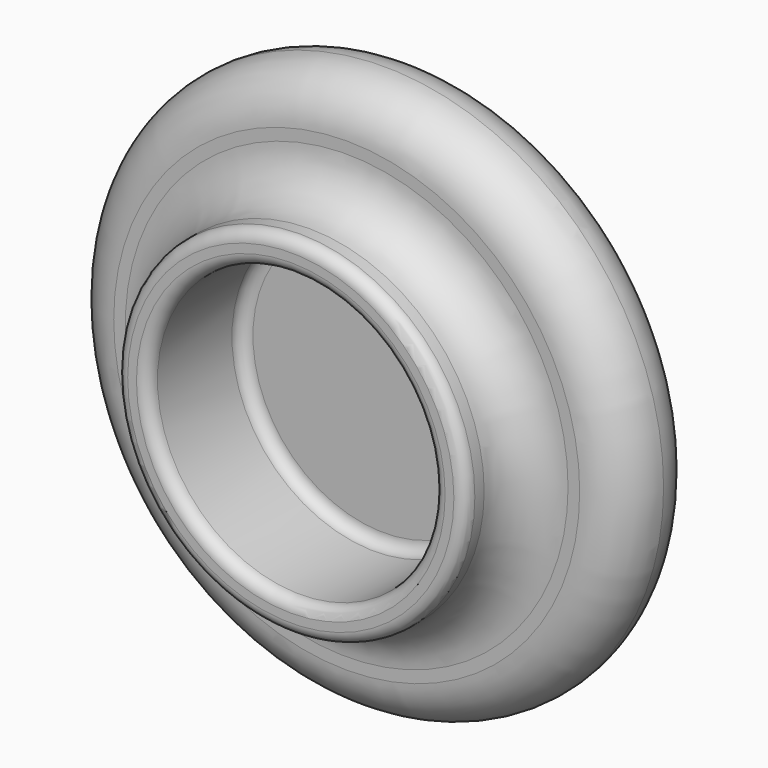
from build123d import *

# Parameters (mm, degrees)
F0_R     = 12
F0_R_2   = 7.5
F0_R_3   = 6.125
F1_DEPTH = 4
F2_DEPTH = 3
F3_DEPTH = 2
F4_R     = 1.99999
F5_R     = 0.5


# Not quite as in the source:
# - a fillet or chamfer is up to 0.001 mm smaller than in the source, because OpenCascade refuses the exact size


with BuildPart() as f1:
    # F0 (on Front) → F1 (new body)
    with BuildSketch(Plane.XZ):
        Circle(F0_R)
        Circle(F0_R_2, mode=Mode.SUBTRACT)
        Circle(F0_R_2)
        Circle(F0_R_3, mode=Mode.SUBTRACT)
        Circle(F0_R_3)
    extrude(amount=-F1_DEPTH)

    # F0 (on Front) → F2 (join)
    with BuildSketch(Plane.XZ):
        Circle(F0_R_2)
        Circle(F0_R_3, mode=Mode.SUBTRACT)
    extrude(amount=F2_DEPTH)

    # F0 (on Front) → F3 (cut)
    with BuildSketch(Plane.XZ):
        Circle(F0_R_3)
    extrude(amount=-F3_DEPTH, mode=Mode.SUBTRACT)

    # F4 (radius 2 in the source; OpenCascade refuses exactly that, so slightly less here)
    f4_edges = [f1.edges().sort_by_distance(p)[0] for p in [
        (-7.5, 0, 0),
        (-12, 0, 0),
        (-12, 4, 0),
    ]]
    fillet(f4_edges, radius=F4_R)

    # F5
    f5_edges = [f1.edges().sort_by_distance(p)[0] for p in [
        (-7.5, -3, 0),
        (-6.125, -3, 0),
        (-6.125, 2, 0),
    ]]
    fillet(f5_edges, radius=F5_R)


solid = f1.part
